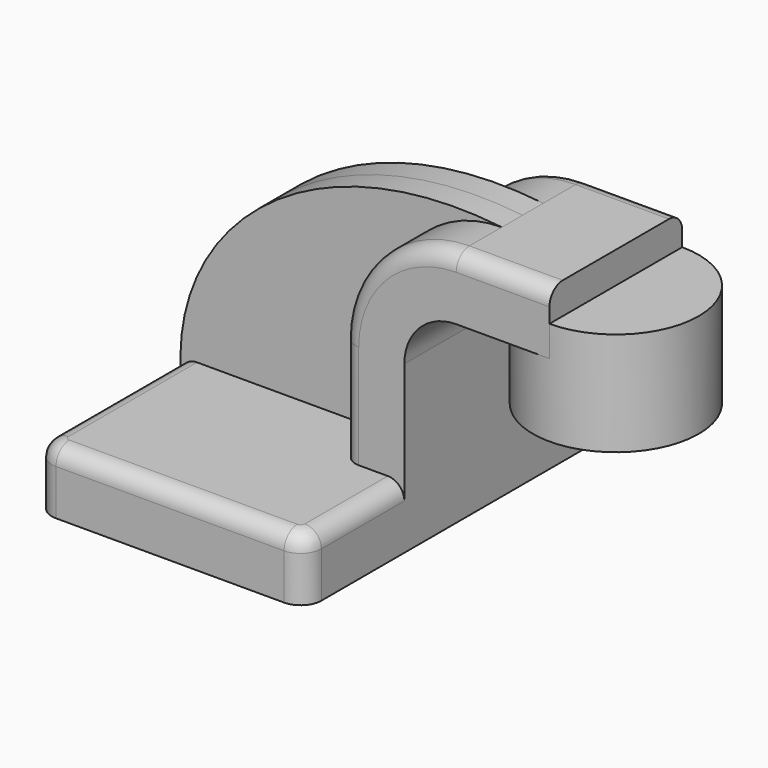
from build123d import *

# Parameters (mm, degrees)
F1_DEPTH     = 63.5
F0_W         = 25.4
F0_H         = 9.398
F2_DEPTH     = 25.4
F3_DEPTH     = 7.9375
F5_R         = 6.35
F6_T1_DEPTH  = 41.275
F6_T3_DEPTH  = 69.85
F6_T5_DEPTH  = 49.2125
F6_T7_DEPTH  = 49.2125
F6_T9_DEPTH  = 31.75
F6_T11_DEPTH = 31.75
F6_T13_DEPTH = 31.877
F6_T16_ANGLE = 90
F6_T18_ANGLE = 90
F6_T20_ANGLE = 90
F6_T22_ANGLE = 90
F6_T24_ANGLE = 90
F6_T26_ANGLE = 90


# Not quite as in the source:
# - a fillet or chamfer that OpenCascade refuses, or shapes differently, is made with other operations: its cross-section is extruded or revolved along the edge and cut away or added


with BuildPart() as f1:
    # F0 (on Front) → F1 (new body, symmetric)
    with BuildSketch(Plane.XZ):
        Polygon((-41.275, 9.525), (-41.275, -9.525), (41.275, -9.525), (41.275, 9.525), (22.225, 9.525), align=None)
    extrude(amount=F1_DEPTH, both=True)

    # F0 (on Front) → F2 (join, symmetric)
    with BuildSketch(Plane.XZ):
        with BuildLine():
            Line((22.225, 9.525), (41.275, 9.525))
            Line((41.275, 9.525), (41.275, 41.402))
            ThreePointArc((41.275, 41.402), (45.9246798487, 52.6273201513), (57.15, 57.277))
            Line((57.15, 57.277), (60.325, 57.277))
            Line((60.325, 57.277), (60.325, 66.675))
            Line((60.325, 66.675), (85.725, 66.675))
            Line((85.725, 66.675), (85.725, 76.327))
            Line((85.725, 76.327), (57.15, 76.327))
            ThreePointArc((57.15, 76.327), (32.4542956671, 66.0977043329), (22.225, 41.402))
            Line((22.225, 41.402), (22.225, 9.525))
        make_face()
        with Locations((73.025, 61.976)):
            Rectangle(F0_W, F0_H)
    extrude(amount=F2_DEPTH, both=True)

    # F0 (on Front) → F3 (join, symmetric)
    with BuildSketch(Plane.XZ):
        with BuildLine():
            add(Edge.make_bspline(
                [(-41.275, 9.525), (-40.9312584529, 49.0607376979), (0, 82.7295482159), (57.15, 76.327)],
                knots=[0, 0, 0, 0, 118.9537213752, 118.9537213752, 118.9537213752, 118.9537213752], degree=3))
            Line((-41.275, 9.525), (22.225, 9.525))
            Line((22.225, 9.525), (22.225, 41.402))
            ThreePointArc((22.225, 41.402), (32.4542956671, 66.0977043329), (57.15, 76.327))
        make_face()
    extrude(amount=F3_DEPTH, both=True)

    # F0 (on Front) → F4 (revolve)
    with BuildSketch(Plane.XZ):
        Polygon((111.125, 66.675), (85.725, 66.675), (85.725, 57.277), (85.725, 34.925), (111.125, 34.925), align=None)
    revolve(axis=Axis((85.725, 0, 55.626), (0, 0, 1)))

    # F5
    f5_edges = [f1.edges().sort_by_distance(p)[0] for p in [
        (41.275, 63.5, 0),
        (-41.275, 63.5, 0),
        (-41.275, -63.5, 0),
        (41.275, -63.5, 0),
    ]]
    fillet(f5_edges, radius=F5_R)

    # F6: fillet of radius 5.08 on 16 edges, made by hand

    # F6_s2 → F6_t1 (cut)
    with BuildSketch(Plane.YZ.offset(57.15)):
        with BuildLine():
            ThreePointArc((25.4, 71.247), (23.9121024484, 74.8391024484), (20.32, 76.327))
            Line((20.32, 76.327), (25.4, 76.327))
            Line((25.4, 76.327), (25.4, 71.247))
        make_face()
        with BuildLine():
            ThreePointArc((-25.4, 71.247), (-23.9121024484, 74.8391024484), (-20.32, 76.327))
            Line((-20.32, 76.327), (-25.4, 76.327))
            Line((-25.4, 76.327), (-25.4, 71.247))
        make_face()
    extrude(amount=F6_T1_DEPTH, mode=Mode.SUBTRACT)

    # F6_s4 → F6_t3 (cut)
    with BuildSketch(Plane.YZ.offset(-34.925)):
        with BuildLine():
            ThreePointArc((-58.42, 9.525), (-62.0121024484, 8.0371024484), (-63.5, 4.445))
            Line((-63.5, 4.445), (-63.5, 9.525))
            Line((-63.5, 9.525), (-58.42, 9.525))
        make_face()
        with BuildLine():
            ThreePointArc((58.42, 9.525), (62.0121024484, 8.0371024484), (63.5, 4.445))
            Line((63.5, 4.445), (63.5, 9.525))
            Line((63.5, 9.525), (58.42, 9.525))
        make_face()
    extrude(amount=F6_T3_DEPTH, mode=Mode.SUBTRACT)

    # F6_s6 → F6_t5 (cut)
    with BuildSketch(Plane.XZ.offset(-57.15)):
        with BuildLine():
            ThreePointArc((-41.275, 4.445), (-39.7871024484, 8.0371024484), (-36.195, 9.525))
            Line((-36.195, 9.525), (-41.275, 9.525))
            Line((-41.275, 9.525), (-41.275, 4.445))
        make_face()
    extrude(amount=F6_T5_DEPTH, mode=Mode.SUBTRACT)

    # F6_s8 → F6_t7 (cut)
    with BuildSketch(Plane.XZ.offset(7.9375)):
        with BuildLine():
            ThreePointArc((-41.275, 4.445), (-39.7871024484, 8.0371024484), (-36.195, 9.525))
            Line((-36.195, 9.525), (-41.275, 9.525))
            Line((-41.275, 9.525), (-41.275, 4.445))
        make_face()
    extrude(amount=F6_T7_DEPTH, mode=Mode.SUBTRACT)

    # F6_s10 → F6_t9 (cut)
    with BuildSketch(Plane.XZ.offset(-57.15)):
        with BuildLine():
            ThreePointArc((36.195, 9.525), (39.7871024484, 8.0371024484), (41.275, 4.445))
            Line((41.275, 4.445), (41.275, 9.525))
            Line((41.275, 9.525), (36.195, 9.525))
        make_face()
    extrude(amount=F6_T9_DEPTH, mode=Mode.SUBTRACT)

    # F6_s12 → F6_t11 (cut)
    with BuildSketch(Plane.XZ.offset(25.4)):
        with BuildLine():
            ThreePointArc((36.195, 9.525), (39.7871024484, 8.0371024484), (41.275, 4.445))
            Line((41.275, 4.445), (41.275, 9.525))
            Line((41.275, 9.525), (36.195, 9.525))
        make_face()
    extrude(amount=F6_T11_DEPTH, mode=Mode.SUBTRACT)

    # F6_s14 → F6_t13 (cut)
    with BuildSketch(Plane.XY.offset(9.525)):
        with BuildLine():
            ThreePointArc((22.225, 20.32), (23.7128975516, 23.9121024484), (27.305, 25.4))
            Line((27.305, 25.4), (22.225, 25.4))
            Line((22.225, 25.4), (22.225, 20.32))
        make_face()
        with BuildLine():
            ThreePointArc((22.225, -20.32), (23.7128975516, -23.9121024484), (27.305, -25.4))
            Line((27.305, -25.4), (22.225, -25.4))
            Line((22.225, -25.4), (22.225, -20.32))
        make_face()
    extrude(amount=F6_T13_DEPTH, mode=Mode.SUBTRACT)

    # F6_s15 → F6_t16 (revolve, cut)
    with BuildSketch(Plane.XZ.offset(-57.15)):
        with BuildLine():
            ThreePointArc((-41.275, 4.445), (-39.7871024484, 8.0371024484), (-36.195, 9.525))
            Line((-36.195, 9.525), (-41.275, 9.525))
            Line((-41.275, 9.525), (-41.275, 4.445))
        make_face()
    revolve(axis=Axis((-34.925, 57.15, 9.525), (0, 0, -1)), revolution_arc=F6_T16_ANGLE, mode=Mode.SUBTRACT)

    # F6_s17 → F6_t18 (revolve, cut)
    with BuildSketch(Plane.XZ.offset(57.15)):
        with BuildLine():
            ThreePointArc((-41.275, 4.445), (-39.7871024484, 8.0371024484), (-36.195, 9.525))
            Line((-36.195, 9.525), (-41.275, 9.525))
            Line((-41.275, 9.525), (-41.275, 4.445))
        make_face()
    revolve(axis=Axis((-34.925, -57.15, 9.525), (0, 0, 1)), revolution_arc=F6_T18_ANGLE, mode=Mode.SUBTRACT)

    # F6_s19 → F6_t20 (revolve, cut)
    with BuildSketch(Plane.YZ.offset(34.925)):
        with BuildLine():
            ThreePointArc((58.42, 9.525), (62.0121024484, 8.0371024484), (63.5, 4.445))
            Line((63.5, 4.445), (63.5, 9.525))
            Line((63.5, 9.525), (58.42, 9.525))
        make_face()
    revolve(axis=Axis((34.925, 57.15, 9.525), (0, 0, -1)), revolution_arc=F6_T20_ANGLE, mode=Mode.SUBTRACT)

    # F6_s21 → F6_t22 (revolve, cut)
    with BuildSketch(Plane.YZ.offset(34.925)):
        with BuildLine():
            ThreePointArc((-58.42, 9.525), (-62.0121024484, 8.0371024484), (-63.5, 4.445))
            Line((-63.5, 4.445), (-63.5, 9.525))
            Line((-63.5, 9.525), (-58.42, 9.525))
        make_face()
    revolve(axis=Axis((34.925, -57.15, 9.525), (0, 0, 1)), revolution_arc=F6_T22_ANGLE, mode=Mode.SUBTRACT)

    # F6_s23 → F6_t24 (revolve, cut)
    with BuildSketch(Plane.YZ.offset(57.15)):
        with BuildLine():
            ThreePointArc((25.4, 71.247), (23.9121024484, 74.8391024484), (20.32, 76.327))
            Line((20.32, 76.327), (25.4, 76.327))
            Line((25.4, 76.327), (25.4, 71.247))
        make_face()
    revolve(axis=Axis((57.15, 25.4, 41.402), (0, -1, 0)), revolution_arc=F6_T24_ANGLE, mode=Mode.SUBTRACT)

    # F6_s25 → F6_t26 (revolve, cut)
    with BuildSketch(Plane.YZ.offset(57.15)):
        with BuildLine():
            ThreePointArc((-25.4, 71.247), (-23.9121024484, 74.8391024484), (-20.32, 76.327))
            Line((-20.32, 76.327), (-25.4, 76.327))
            Line((-25.4, 76.327), (-25.4, 71.247))
        make_face()
    revolve(axis=Axis((57.15, -25.4, 41.402), (0, -1, 0)), revolution_arc=F6_T26_ANGLE, mode=Mode.SUBTRACT)


solid = f1.part
